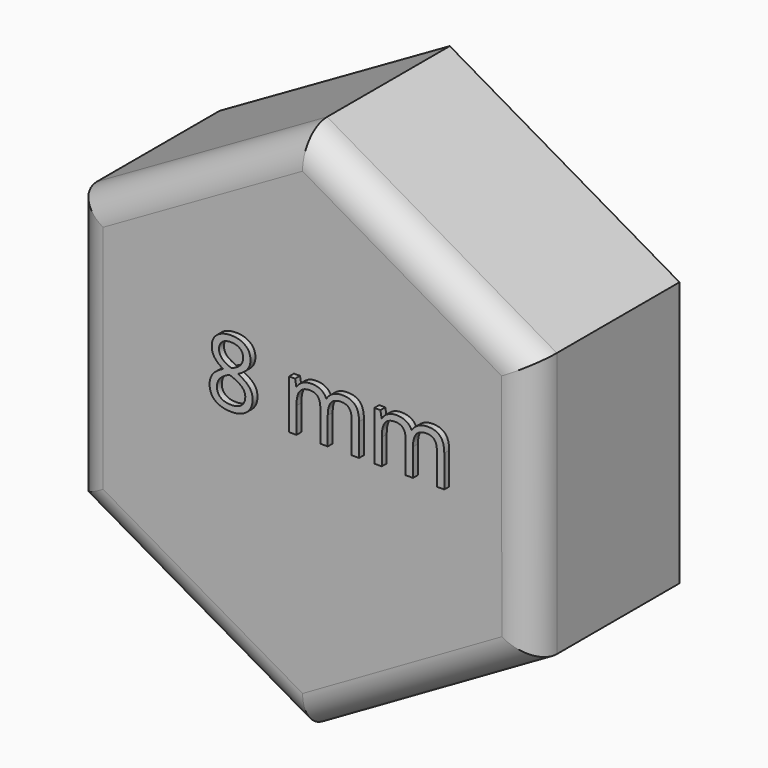
from build123d import *

# Parameters (mm, degrees)
F3_DEPTH     = 6
F4_R         = 1
F5_TEXT_SIZE = 2.9899556178
F6_DEPTH     = 0.2


# Not quite as in the source:
# - Text() gives the source's letters only with a copy of the font that has no kerning and outlines rounded to 1/6400 em; it was checked with that copy


with BuildPart() as f3:
    # F2 (on Front) → F3 (new body)
    with BuildSketch(Plane.XZ):
        Polygon((7.4963159859, -4.3287435547), (7.4915997684, 4.3125804514), (0, 8.6566042155), (-7.5077288784, 4.3566742212), (-7.5077288784, -4.3242308311), (0, -8.6466483772), align=None)
    extrude(amount=F3_DEPTH)

    # F4
    f4_edges = [f3.edges().sort_by_distance(p)[0] for p in [
        (3.7458, -6, 6.484592),
        (-3.753864, -6, 6.506639),
        (-7.507729, -6, 0.016222),
        (-3.753864, -6, -6.48544),
        (3.748158, -6, -6.487696),
        (7.493958, -6, -0.008082),
    ]]
    fillet(f4_edges, radius=F4_R)

    # F5 (on face) → F6 (join)
    with BuildSketch(Plane.XZ.offset(6)):
        with Locations((-3.0258864782, 0)):
            Text('8 mm', F5_TEXT_SIZE, font='Open Sans', text_align=(TextAlign.LEFT, TextAlign.BOTTOM))
    extrude(amount=F6_DEPTH)


solid = f3.part
